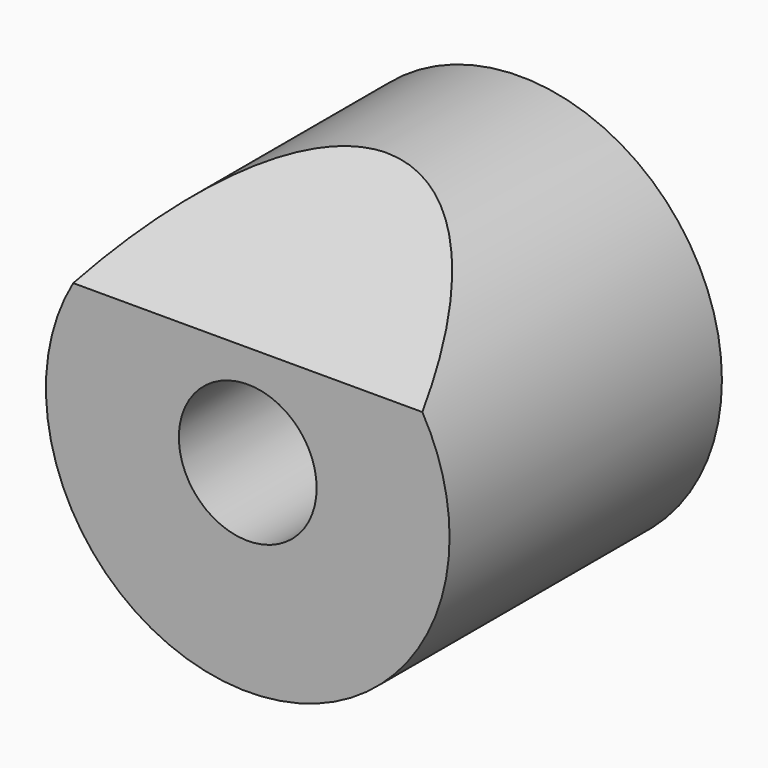
from build123d import *

# Parameters (mm, degrees)
F0_R     = 12.45
F0_R_2   = 4.25
F1_DEPTH = 21
F3_DEPTH = 12.5


with BuildPart() as f1:
    # F0 (on Front) → F1 (new body)
    with BuildSketch(Plane.XZ):
        Circle(F0_R)
        Circle(F0_R_2, mode=Mode.SUBTRACT)
    extrude(amount=F1_DEPTH)

    # F2 (on Right) → F3 (cut, symmetric)
    with BuildSketch(Plane.YZ):
        Polygon((-10.2612849931, 12.45), (-21, 12.45), (-21, 6.25), align=None)
    extrude(amount=F3_DEPTH, both=True, mode=Mode.SUBTRACT)


solid = f1.part
